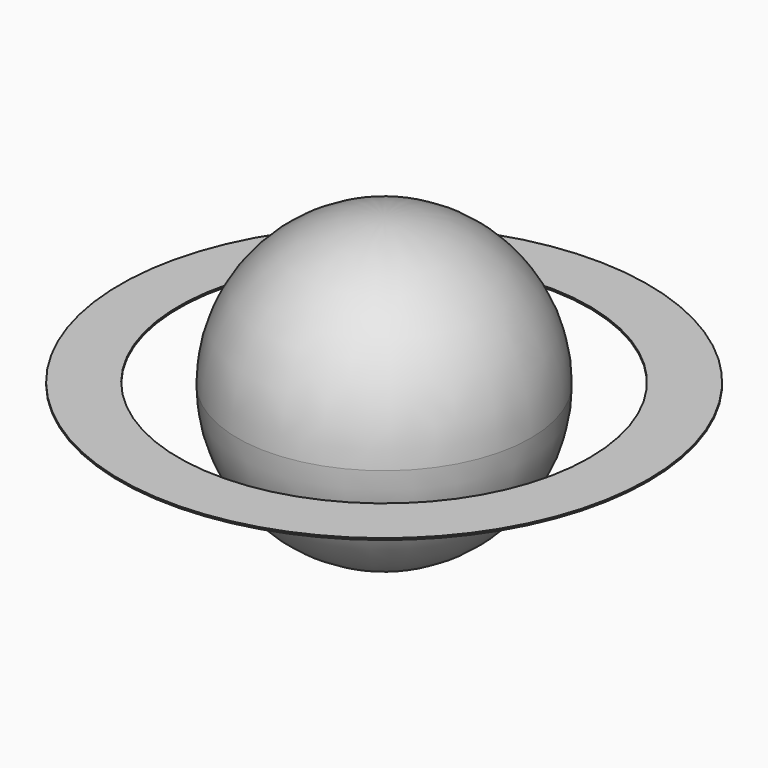
from build123d import *

# Parameters (mm, degrees)
F0_R     = 63.5
F1_DEPTH = 63.5
F2_DEPTH = 63.5
F3_R     = 63.49999
F4_R     = 114.3
F4_R_2   = 88.9
F5_DEPTH = 0.762


# Not quite as in the source:
# - a fillet or chamfer is up to 0.001 mm smaller than in the source, because OpenCascade refuses the exact size


with BuildPart() as f1:
    # F0 (on Top) → F1 (new body)
    with BuildSketch(Plane.XY):
        Circle(F0_R)
    extrude(amount=F1_DEPTH)

    # F2 (add): a face of the model
    f2_faces = [f1.faces().sort_by_distance(p)[0] for p in [
        (0, 0, 0),
    ]]
    extrude(f2_faces, amount=F2_DEPTH)

    # F3 (radius 63.5 in the source; OpenCascade refuses exactly that, so slightly less here)
    f3_edges = [f1.edges().sort_by_distance(p)[0] for p in [
        (63.5, 0, 31.75),
        (-63.5, 0, 0),
        (-63.5, 0, 63.5),
        (63.5, 0, -31.75),
        (-63.5, 0, -63.5),
    ]]
    fillet(f3_edges, radius=F3_R)


with BuildPart() as f5:
    # F4 (on Top) → F5 (new body)
    with BuildSketch(Plane.XY):
        Circle(F4_R)
        Circle(F4_R_2, mode=Mode.SUBTRACT)
    extrude(amount=F5_DEPTH)


solid = Compound([f1.part, f5.part])
